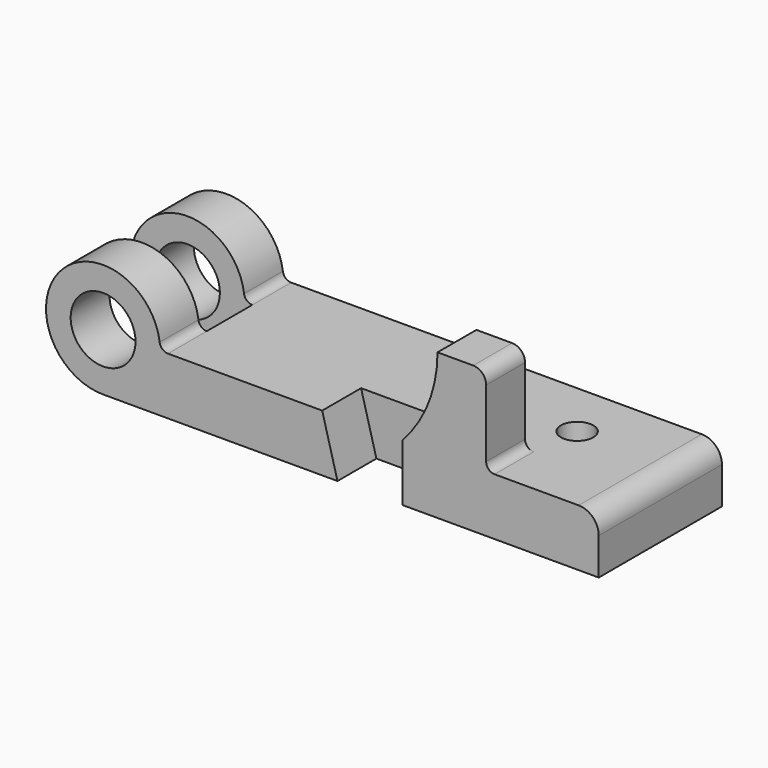
from build123d import *

# Parameters (mm, degrees)
F1_DEPTH      = 30.1625
F1_DEPTH_BACK = 30.1625
F2_DEPTH      = 11.1125
F2_DEPTH_BACK = 30.1625
F0_R          = 12.7
F3_DEPTH      = 30.1625
F3_DEPTH_BACK = 30.1625
F4_W          = 41.275
F4_H          = 34.798
F5_DEPTH      = 38.1
F6_W          = 11.1633
F6_H          = 50.8
F7_DEPTH      = 25.4
F7_DEPTH_BACK = 25.4
F8_R          = 6.35
F9_DEPTH      = 25.4
F10_R         = 7.874
F11_R         = 5.08
F12_F1_R      = 3.302
F12_F2_R      = 3.302


with BuildPart() as f1:
    # F0 (on Front) → F1 (new body, two sides)
    with BuildSketch(Plane.XZ) as f1_sk:
        with BuildLine():
            ThreePointArc((131.0386, 34.798), (127.4644153616, 16.0823576341), (117.2464, 0))
            Line((117.2464, 0), (117.2464, -22.352))
            Line((117.2464, -22.352), (194.2084, -22.352))
            Line((194.2084, -22.352), (194.2084, 0))
            Line((194.2084, 0), (150.0886, 0))
            Line((150.0886, 0), (150.0886, 34.798))
            Line((150.0886, 34.798), (131.0386, 34.798))
        make_face()
    extrude(amount=-F1_DEPTH)
    extrude(f1_sk.sketch, amount=F1_DEPTH_BACK)

    # F0 (on Front) → F2 (join, two sides)
    with BuildSketch(Plane.XZ) as f2_sk:
        Polygon((117.2464, 0), (85.852, 0), (91.8464, -22.352), (117.2464, -22.352), align=None)
    extrude(amount=F2_DEPTH)
    extrude(f2_sk.sketch, amount=-F2_DEPTH_BACK)

    # F0 (on Front) → F3 (join, two sides)
    with BuildSketch(Plane.XZ) as f3_sk:
        with BuildLine():
            Line((85.852, 0), (22.352, 0))
            ThreePointArc((22.352, 0), (15.8052507731, -15.8052507731), (0, -22.352))
            Line((0, -22.352), (91.8464, -22.352))
            Line((91.8464, -22.352), (85.852, 0))
        make_face()
        with BuildLine():
            ThreePointArc((0, -22.352), (15.8052507731, -15.8052507731), (22.352, 0))
            ThreePointArc((22.352, 0), (-15.8052507731, 15.8052507731), (0, -22.352))
        make_face()
        Circle(F0_R, mode=Mode.SUBTRACT)
    extrude(amount=F3_DEPTH)
    extrude(f3_sk.sketch, amount=-F3_DEPTH_BACK)

    # F4 (on face) → F5 (cut)
    with BuildSketch(Plane.YZ.offset(150.0886)):
        with Locations((9.525, 17.399)):
            Rectangle(F4_W, F4_H)
    extrude(amount=-F5_DEPTH, mode=Mode.SUBTRACT)

    # F6 (on Right) → F7 (cut, two sides)
    with BuildSketch(Plane.YZ) as f7_sk:
        with Locations((5.58165, 25.4)):
            Rectangle(F6_W, F6_H)
        with Locations((-5.58165, 25.4)):
            Rectangle(F6_W, F6_H)
        Polygon((11.1633, 0), (0, 0), (-11.1633, 0), (-11.1633, -23.6136056483), (11.1633, -23.6136056483), align=None)
    extrude(amount=-F7_DEPTH, mode=Mode.SUBTRACT)
    extrude(f7_sk.sketch, amount=F7_DEPTH_BACK, mode=Mode.SUBTRACT)

    # F8 (on face) → F9 (cut)
    with BuildSketch(Plane.XY):
        with Locations((155.3464, 7.8105)):
            Circle(F8_R)
    extrude(amount=-F9_DEPTH, mode=Mode.SUBTRACT)

    # F10
    f10_edges = [f1.edges().sort_by_distance(p)[0] for p in [
        (194.2084, 0, 0),
    ]]
    fillet(f10_edges, radius=F10_R)

    # F11
    f11_edges = [f1.edges().sort_by_distance(p)[0] for p in [
        (150.0886, -20.6375, 34.798),
    ]]
    fillet(f11_edges, radius=F11_R)

    # F12: fillet of radius 3.302 on 3 edges, made by hand

    # F12_f1
    f12_f1_edges = [f1.edges().sort_by_distance(p)[0] for p in [
        (150.0886, -20.6375, 0),
    ]]
    fillet(f12_f1_edges, radius=F12_F1_R)

    # F12_f2
    f12_f2_edges = [f1.edges().sort_by_distance(p)[0] for p in [
        (22.352, 20.6629, 0),
    ]]
    fillet(f12_f2_edges, radius=F12_F2_R)


solid = f1.part
